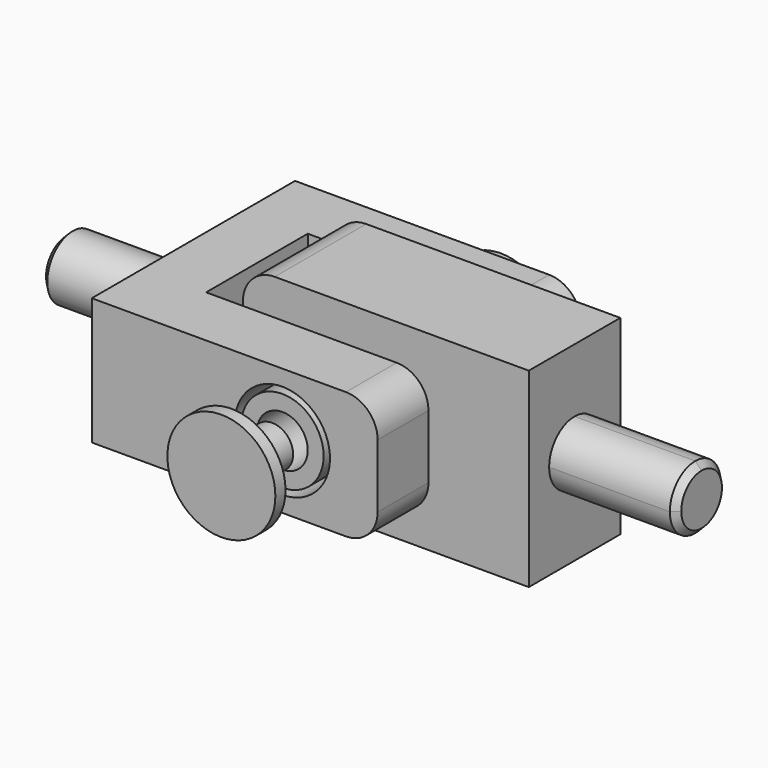
from build123d import *

# Parameters (mm, degrees)
F0_R          = 5
F1_DEPTH      = 20
F3_DEPTH      = 20
F4_R          = 5
F6_D          = 15
F7_SIZE       = 1
F5_R          = 6.5
F5_R_2        = 4
F8_DEPTH      = 40
F8_DEPTH_BACK = 1
F9_START      = 11
F5_R_3        = 7.5
F9_DEPTH      = 18
F10_R         = 5
F11_START     = 15
F5_W          = 20
F5_H          = 10
F11_DEPTH     = 10
F12_R         = 4.99999
F13_SIZE      = 1
F15_START     = -1
F14_R         = 8.5
F15_DEPTH     = 2
F16_START     = -8
F16_DEPTH     = 2
F5_R_4        = 3.3
F18_DEPTH     = 30
F19_START     = 42
F19_DEPTH     = 8


# Not quite as in the source:
# - a fillet or chamfer is up to 0.001 mm smaller than in the source, because OpenCascade refuses the exact size
# - a feature names something its author has since deleted; it is built from what else it names


with BuildPart() as f1:
    # F0 (on Right) → F1 (new body)
    with BuildSketch(Plane.YZ):
        with Locations((-20, -10)):
            Circle(F0_R)
    extrude(amount=-F1_DEPTH)

    # F2 (on Top) → F3 (join)
    with BuildSketch(Plane.XY):
        Polygon((45, 0), (0, 0), (0, -40), (45, -40), (45, -30), (15, -30), (10, -30), (10, -10), (15, -10), (45, -10), align=None)
    extrude(amount=-F3_DEPTH)

    # F4
    f4_edges = [f1.edges().sort_by_distance(p)[0] for p in [
        (45, -35, 0),
        (45, -5, 0),
        (45, -35, -20),
        (45, -5, -20),
    ]]
    fillet(f4_edges, radius=F4_R)

    # F6 (through all)
    with Locations(Plane(origin=(0, 0, 0), x_dir=(1, 0, 0), z_dir=(0, 1, 0))):
        with Locations((30, 10)):
            Hole(F6_D / 2)

    # F7
    f7_edges = [f1.edges().sort_by_distance(p)[0] for p in [
        (-20, -25, -10),
    ]]
    chamfer(f7_edges, length=F7_SIZE)


with BuildPart() as f8:
    # F5 (on Front) → F8 (new body, two sides)
    with BuildSketch(Plane.XZ) as f8_sk:
        with Locations((30, -10)):
            Circle(F5_R)
        with Locations((30, -10)):
            Circle(F5_R_2, mode=Mode.SUBTRACT)
    extrude(amount=F8_DEPTH)
    extrude(f8_sk.sketch, amount=-F8_DEPTH_BACK)

    # F14 (on Front) → F15 (join)
    with BuildSketch(Plane.XZ.offset(F15_START)):
        with Locations((30, -10)):
            Circle(F14_R)
    extrude(amount=-F15_DEPTH)

    # F5 (on Front) → F18 (join)
    with BuildSketch(Plane.XZ):
        with Locations((30, -10)):
            Circle(F5_R_2)
        with Locations((30, -10)):
            Circle(F5_R_4, mode=Mode.SUBTRACT)
        with Locations((30, -10)):
            Circle(F5_R_4)
    extrude(amount=F18_DEPTH)


with BuildPart() as f9:
    # F5 (on Front) → F9 (new body)
    with BuildSketch(Plane.XZ.offset(F9_START)):
        Polygon((60, 5), (15, 5), (15, -25), (60, -25), (60, -15), (60, -5), align=None)
        with Locations((30, -10)):
            Circle(F5_R_3, mode=Mode.SUBTRACT)
    extrude(amount=F9_DEPTH)

    # F10
    f10_edges = [f9.edges().sort_by_distance(p)[0] for p in [
        (15, -20, 5),
        (15, -20, -25),
    ]]
    fillet(f10_edges, radius=F10_R)

    # F5 (on Front) → F11 (join)
    with BuildSketch(Plane.XZ.offset(F11_START)):
        with Locations((70, -10)):
            Rectangle(F5_W, F5_H)
    extrude(amount=F11_DEPTH)

    # F12 (radius 5 in the source; OpenCascade refuses exactly that, so slightly less here)
    f12_edges = [f9.edges().sort_by_distance(p)[0] for p in [
        (70, -25, -5),
        (70, -15, -5),
        (70, -15, -15),
        (70, -25, -15),
    ]]
    fillet(f12_edges, radius=F12_R)

    # F13
    f13_edges = [f9.edges().sort_by_distance(p)[0] for p in [
        (80, -20, -15),
        (80, -16.464463, -13.535537),
        (80, -23.535537, -13.535537),
        (80, -15, -10),
        (80, -25, -10),
        (80, -16.464463, -6.464463),
        (80, -23.535537, -6.464463),
        (80, -20, -5),
    ]]
    chamfer(f13_edges, length=F13_SIZE)


with BuildPart() as f16:
    # F14 (on Front) → F16 (new body)
    with BuildSketch(Plane.XZ.offset(F16_START)):
        with Locations((30, -10)):
            Circle(F14_R)
    extrude(amount=-F16_DEPTH)


with BuildPart() as f16_1:
    # F17: moved
    add(f16.part.moved(Location((0, -60, 0))))

    # F5 (on Front) → F19 (join)
    with BuildSketch(Plane.XZ.offset(F19_START)):
        with Locations((30, -10)):
            Circle(F5_R_4)
    extrude(amount=F19_DEPTH)


solid = Compound([f1.part, f8.part, f9.part, f16_1.part])
